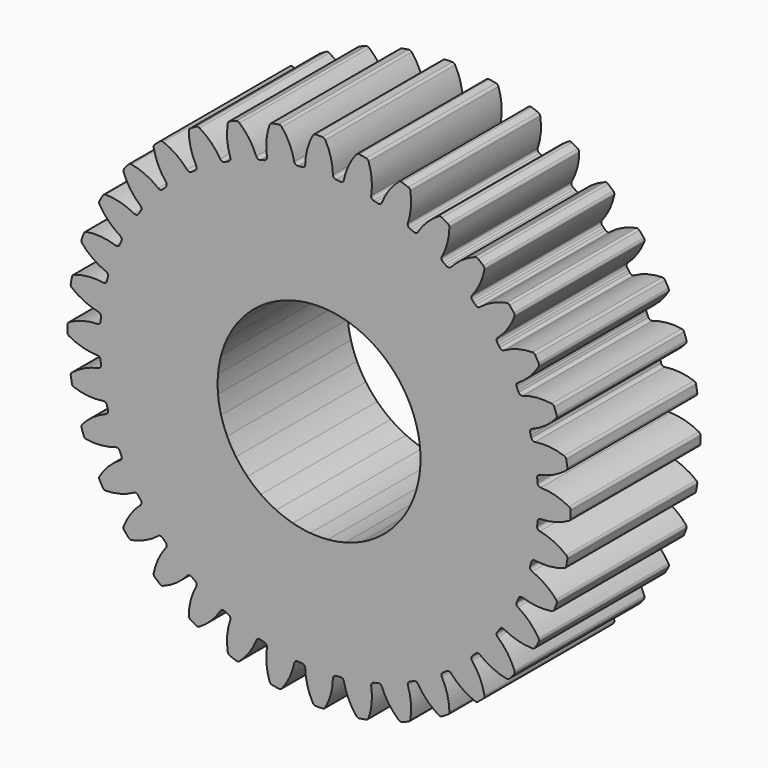
from build123d import *

# Parameters (mm, degrees)
F1_DEPTH = 40
F2_R     = 0.8
F3_COUNT = 36


with BuildPart() as f1:
    # F0 (on Front) → F1 (new body)
    with BuildSketch(Plane.XZ):
        with BuildLine():
            ThreePointArc((-2.1788935687, 24.9048674523), (0, 25), (2.1788935687, 24.9048674523))
            Line((2.1788935687, 24.9048674523), (4.7064101084, 53.794513697))
            ThreePointArc((4.7064101084, 53.794513697), (4.0584956143, 53.8472711783), (3.4099929772, 53.892225301))
            ThreePointArc((3.4099929772, 53.892225301), (2.930615325, 58.0893505196), (1.3, 61.9863694694))
            ThreePointArc((1.3, 61.9863694694), (0, 62), (-1.3, 61.9863694694))
            ThreePointArc((-1.3, 61.9863694694), (-2.930615325, 58.0893505196), (-3.4099929772, 53.892225301))
            ThreePointArc((-3.4099929772, 53.892225301), (-4.0584956143, 53.8472711783), (-4.7064101084, 53.794513697))
            Line((-4.7064101084, 53.794513697), (-2.1788935687, 24.9048674523))
        make_face()
    extrude(amount=F1_DEPTH)

    # F2
    f2_edges = [f1.edges().sort_by_distance(p)[0] for p in [
        (-3.409993, -20, 53.892225),
        (-1.3, -20, 61.986369),
        (1.3, -20, 61.986369),
        (3.409993, -20, 53.892225),
    ]]
    fillet(f2_edges, radius=F2_R)

    # F3: F1 ×36 about axis
    f3_axis = Axis((0, 0, 0), (0, 1, 0))


with BuildPart() as f1_1:
    add(f1.part)
    for i in range(1, F3_COUNT):
        add(f1.part.rotate(f3_axis, i * 360 / F3_COUNT))


solid = f1_1.part
